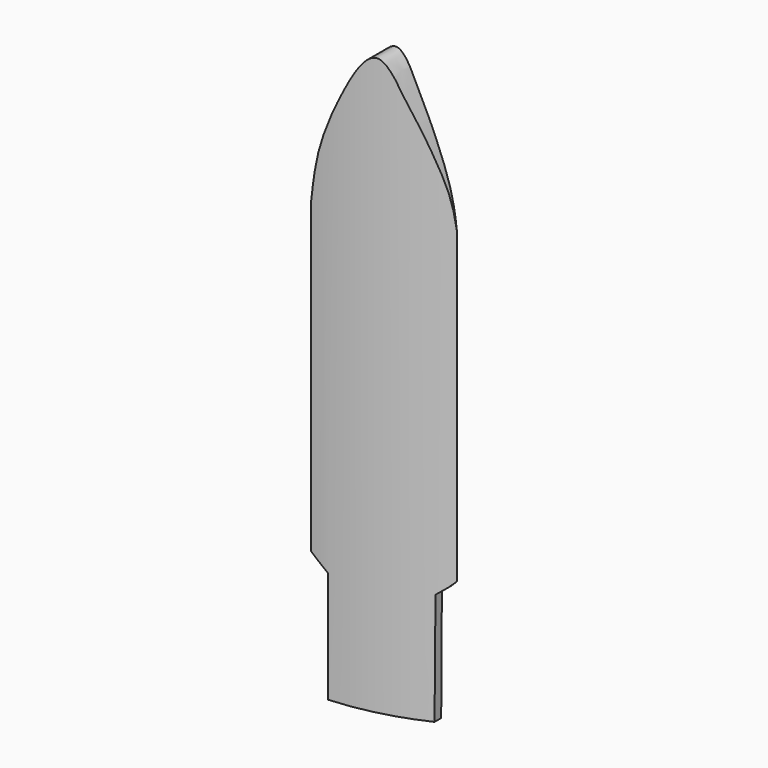
from build123d import *

# Parameters (mm, degrees)
F2_DEPTH    = 3.556
F3_T1_DEPTH = 100.1960824302


# Not quite as in the source:
# - a fillet or chamfer that OpenCascade refuses, or shapes differently, is made with other operations: its cross-section is extruded or revolved along the edge and cut away or added


with BuildPart() as f2:
    # F1 (on offset) → F2 (new body)
    with BuildSketch(Plane.XZ.offset(-3.556)):
        with BuildLine():
            Line((-4.7608385794, 30.2790850401), (-4.7608385794, -3.7161211949))
            Line((-4.7608385794, -3.7161211949), (-2.9770701658, -5.2399407141))
            Line((-2.9770701658, -5.2399407141), (-2.9770701658, -17.5244603306))
            Line((-2.9770701658, -17.5244603306), (6.7130425275, -17.5824380662))
            Line((6.7130425275, -17.5824380662), (6.7868899709, -5.2399407141))
            Line((6.7868899709, -5.2399407141), (7.8166099265, -4.4050700963))
            Line((7.8166099265, -4.4050700963), (8.4343710914, -3.7950705737))
            Line((8.4343710914, -3.7950705737), (8.4343710914, 30.2790850401))
            add(Edge.make_bspline(
                [(-4.7608385794, 30.2790850401), (-4.5736827726, 31.9597863049), (-4.1702659217, 35.5825604162), (-1.8450394854, 41.296641728), (1.8526726795, 48.0701768841), (4.4004372394, 42.0002992607), (5.4469394771, 40.1971389087), (7.9610301665, 34.2093633894), (8.287935143, 31.4949825195), (8.4343710914, 30.2790850401)],
                knots=[0, 0, 0, 0, 0.1477315981, 0.3184374406, 0.4674111086, 0.6017993168, 0.7078404462, 0.869128143, 1, 1, 1, 1], degree=3))
        make_face()
    extrude(amount=F2_DEPTH)

    # F3: fillet of radius 26.3680405282 on 1 edges, made by hand

    # F3_s2 → F3_t1 (cut)
    with BuildSketch(Plane.XY.offset(-36.8560339819)):
        with BuildLine():
            ThreePointArc((8.4343710914, 3.556), (2.057056347, 0.904513961), (-4.7900142719, 0))
            Line((-4.7900142719, 0), (-4.7900142719, -0.5273608106))
            Line((-4.7900142719, -0.5273608106), (8.4343710914, -0.5273608106))
            Line((8.4343710914, -0.5273608106), (8.961731902, 0))
            ThreePointArc((8.961731902, 0), (8.961731902, 1.778), (8.6988587987, 3.0997591894))
            Line((8.6988587987, 3.0997591894), (8.4343710914, 3.556))
        make_face()
    extrude(amount=F3_T1_DEPTH, mode=Mode.SUBTRACT)


solid = f2.part
